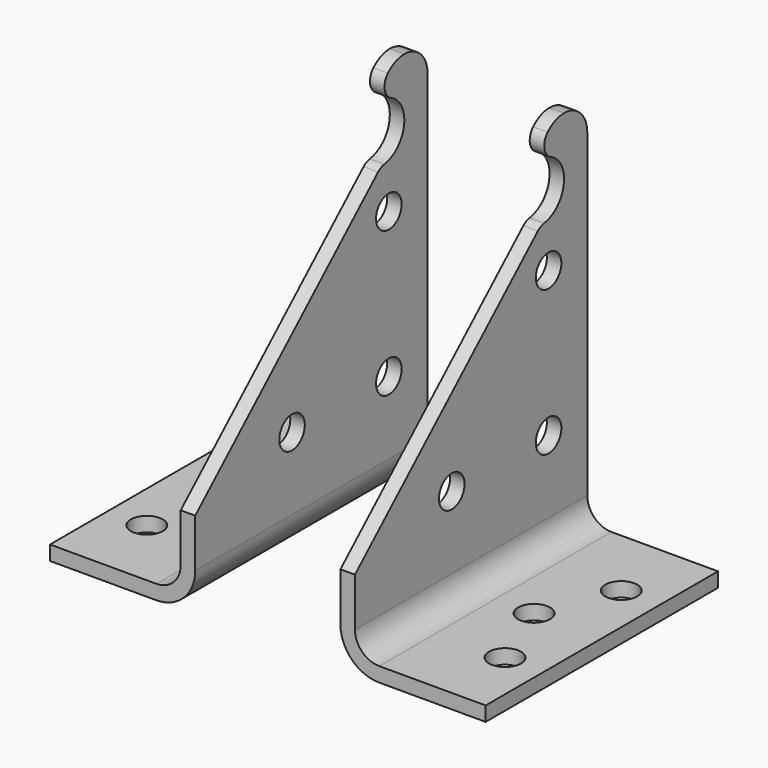
from build123d import *

# Parameters (mm, degrees)
F1_DEPTH = 60
F3_DEPTH = 25
F4_R     = 3
F6_D     = 6.6
F8_D     = 6.6


# Not quite as in the source:
# - a feature names something its author has since deleted; it is built from what else it names


with BuildPart() as f1:
    # F0 (on Front) → F1 (new body)
    with BuildSketch(Plane.XZ):
        with BuildLine():
            ThreePointArc((-23, 0), (-17.3431457505, 2.3431457505), (-15, 8))
            Line((-15, 8), (-15, 80))
            Line((-15, 80), (-18, 80))
            Line((-18, 80), (-18, 8))
            ThreePointArc((-18, 8), (-19.4644660941, 4.4644660941), (-23, 3))
            Line((-23, 3), (-45, 3))
            Line((-45, 3), (-45, 0))
            Line((-45, 0), (-23, 0))
        make_face()
    extrude(amount=F1_DEPTH)

    # F2 (on face) → F3 (cut)
    with BuildSketch(Plane(origin=(-18, 0, 0), x_dir=(0, -1, 0), z_dir=(-1, 0, 0))):
        with BuildLine():
            Line((60, 18), (60, 80))
            Line((60, 80), (6.0000000167, 80))
            ThreePointArc((6.0000000167, 80), (10.242640693, 78.2426406812), (12, 74))
            ThreePointArc((12, 74), (6, 68), (12, 62))
            Line((12, 62), (60, 18))
        make_face()
        with BuildLine():
            ThreePointArc((0, 74), (1.7573593188, 78.242640693), (6.0000000167, 80))
            Line((6.0000000167, 80), (0, 80))
            Line((0, 80), (0, 74))
        make_face()
    extrude(amount=-F3_DEPTH, mode=Mode.SUBTRACT)

    # F4
    f4_edges = [f1.edges().sort_by_distance(p)[0] for p in [
        (-16.5, -12, 74),
        (-16.5, -12, 62),
    ]]
    fillet(f4_edges, radius=F4_R)

    # F6 (through all)
    with Locations(Plane(origin=(0, 0, 0), x_dir=(1, 0, 0), z_dir=(0, 0, -1))):
        with Locations((-37, 15), (-31, 30), (-37, 45)):
            Hole(F6_D / 2)

    # F8 (through all)
    with Locations(Plane(origin=(-18, 0, 0), x_dir=(0, -1, 0), z_dir=(-1, 0, 0))):
        with Locations((10, 53), (10, 23), (35, 23)):
            Hole(F8_D / 2)


with BuildPart() as f9_1:
    # F9: instance of F1
    add(f1.part.mirror(Plane.YZ))


solid = Compound([f1.part, f9_1.part])
